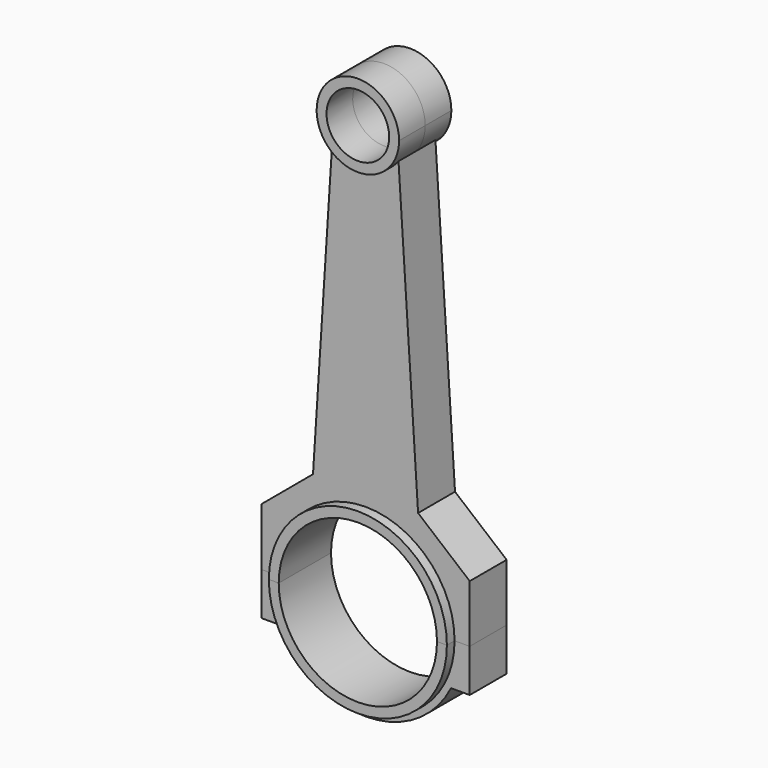
from build123d import *

# Parameters (mm, degrees)
F1_DEPTH = 12.5857
F2_DEPTH = 12.5857
F3_DEPTH = 8.89
F4_DEPTH = 12.5857
F5_DEPTH = 8.89


with BuildPart() as f1:
    # F0 (on Front) → F1 (new body, symmetric)
    with BuildSketch(Plane.XZ):
        with BuildLine():
            Line((30.48, 0), (34.29, 0))
            ThreePointArc((34.29, 0), (0, 34.29), (-34.29, 0))
            Line((-34.29, 0), (-30.48, 0))
            ThreePointArc((-30.48, 0), (0, 30.48), (30.48, 0))
        make_face()
    extrude(amount=F1_DEPTH, both=True)



with BuildPart() as f2:
    # F0 (on Front) → F2 (new body, symmetric)
    with BuildSketch(Plane.XZ):
        with BuildLine():
            ThreePointArc((12.0399923395, 165.876408053), (12.0587464642, 165.4884053449), (12.065, 165.1))
            ThreePointArc((12.065, 165.1), (-0.3884053449, 153.0412535358), (-12.0399923395, 165.876408053))
            Line((-12.0399923395, 165.876408053), (-12.7039469543, 155.5802648785))
            ThreePointArc((-12.7039469543, 155.5802648785), (0, 149.225), (12.7039469543, 155.5802648785))
            Line((12.7039469543, 155.5802648785), (12.0399923395, 165.876408053))
        make_face()
        with BuildLine():
            ThreePointArc((-12.0399923395, 165.876408053), (0, 177.165), (12.0399923395, 165.876408053))
            Line((12.0399923395, 165.876408053), (12.7039469543, 155.5802648785))
            ThreePointArc((12.7039469543, 155.5802648785), (15.0613874344, 160.0830055262), (15.875, 165.1))
            ThreePointArc((15.875, 165.1), (-5.0169944738, 180.1613874344), (-12.7039469543, 155.5802648785))
            Line((-12.7039469543, 155.5802648785), (-12.0399923395, 165.876408053))
        make_face()
    extrude(amount=F2_DEPTH, both=True)


with BuildPart() as f1_1:
    add(f1.part)

    add(f2.part)  # F3 merges F2
    # F0 (on Front) → F3 (join, symmetric)
    with BuildSketch(Plane.XZ):
        with BuildLine():
            Line((20.2382598072, 38.7434177101), (12.7039469543, 155.5802648785))
            ThreePointArc((12.7039469543, 155.5802648785), (0, 149.225), (-12.7039469543, 155.5802648785))
            Line((-12.7039469543, 155.5802648785), (-20.2382598072, 38.7434177101))
            Line((-20.2382598072, 38.7434177101), (-40.132, 22.128129378))
            Line((-40.132, 22.128129378), (-40.132, 0))
            Line((-40.132, 0), (-34.29, 0))
            ThreePointArc((-34.29, 0), (0, 34.29), (34.29, 0))
            Line((34.29, 0), (40.132, 0))
            Line((40.132, 0), (40.132, 22.128129378))
            Line((40.132, 22.128129378), (20.2382598072, 38.7434177101))
        make_face()
    extrude(amount=F3_DEPTH, both=True)


with BuildPart() as f4:
    # F0 (on Front) → F4 (new body, symmetric)
    with BuildSketch(Plane.XZ):
        with BuildLine():
            ThreePointArc((-34.29, 0), (0, -34.29), (34.29, 0))
            Line((34.29, 0), (30.48, 0))
            ThreePointArc((30.48, 0), (0, -30.48), (-30.48, 0))
            Line((-30.48, 0), (-34.29, 0))
        make_face()
    extrude(amount=F4_DEPTH, both=True)

    # F0 (on Front) → F5 (join, symmetric)
    with BuildSketch(Plane.XZ):
        with BuildLine():
            Line((40.132, -16.51), (40.132, 0))
            Line((40.132, 0), (34.29, 0))
            ThreePointArc((34.29, 0), (0, -34.29), (-34.29, 0))
            Line((-34.29, 0), (-40.132, 0))
            Line((-40.132, 0), (-40.132, -16.51))
            Line((-40.132, -16.51), (-32.9221627479, -16.51))
            ThreePointArc((-32.9221627479, -16.51), (0, -36.83), (32.9221627479, -16.51))
            Line((32.9221627479, -16.51), (40.132, -16.51))
        make_face()
    extrude(amount=F5_DEPTH, both=True)


solid = Compound([f1_1.part, f4.part])
